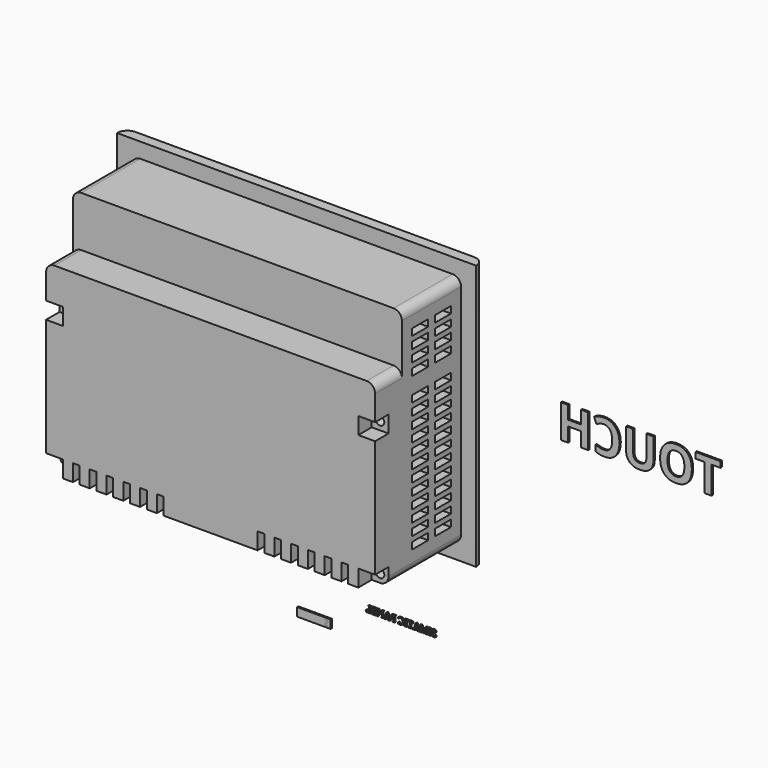
from build123d import *

# Parameters (mm, degrees)
F0_W          = 214
F0_H          = 158
F1_DEPTH      = 6.2
F2_W          = 196
F2_H          = 140
F3_DEPTH      = 44
F5_DEPTH      = 158
F6_W          = 196
F6_H          = 110
F7_DEPTH      = 20
F8_R          = 5
F9_W          = 12
F9_H          = 4
F10_DEPTH     = 10
F11_W         = 12
F11_H         = 4
F12_DEPTH     = 10
F13_W         = 10
F13_H         = 10
F14_DEPTH     = 10
F15_R         = 2.5
F16_DEPTH     = 20
F17_W         = 160
F17_H         = 120
F18_DEPTH     = 2
F19_W         = 140
F19_H         = 80
F20_DEPTH     = 2
F21_W         = 140
F21_H         = 80
F22_DEPTH     = 2
F23_W         = 4
F23_H         = 12
F24_DEPTH     = 10
F25_TEXT_SIZE = 5.5555555556
F26_DEPTH     = 1
F27_TEXT_SIZE = 27.7777777778
F28_DEPTH     = 1
F29_TEXT_SIZE = 4.1666666667
F30_DEPTH     = 1
F31_W         = 20
F31_H         = 5
F32_DEPTH     = 1


# Not quite as in the source:
# - Text() gives the source's letters only with a copy of the font that has no kerning and outlines rounded to 1/6400 em; it was checked with that copy


with BuildPart() as f1:
    # F0 (on Front) → F1 (new body)
    with BuildSketch(Plane.XZ):
        Rectangle(F0_W, F0_H)
    extrude(amount=-F1_DEPTH)

    # F2 (on face) → F3 (join)
    with BuildSketch(Plane.XZ):
        Rectangle(F2_W, F2_H)
    extrude(amount=F3_DEPTH)

    # F4 (on face) → F5 (cut)
    with BuildSketch(Plane.XY.offset(79)):
        with BuildLine():
            Line((107, 6.2), (100.8, 6.2))
            ThreePointArc((100.8, 6.2), (105.1840620434, 4.3840620434), (107, 0))
            Line((107, 0), (107, 6.2))
        make_face()
        with BuildLine():
            ThreePointArc((-107, 0), (-105.1840620434, 4.3840620434), (-100.8, 6.2))
            Line((-100.8, 6.2), (-107, 6.2))
            Line((-107, 6.2), (-107, 0))
        make_face()
    extrude(amount=-F5_DEPTH, mode=Mode.SUBTRACT)

    # F6 (on face) → F7 (join)
    with BuildSketch(Plane.XZ.offset(44)):
        with Locations((0, -15)):
            Rectangle(F6_W, F6_H)
    extrude(amount=F7_DEPTH)

    # F8
    f8_edges = [f1.edges().sort_by_distance(p)[0] for p in [
        (-98, -32, -70),
        (98, -32, -70),
        (98, -22, 70),
        (98, -54, 40),
        (-98, -22, 70),
        (-98, -54, 40),
    ]]
    fillet(f8_edges, radius=F8_R)

    # F9 (on face) → F10 (cut)
    with BuildSketch(Plane(origin=(-98, 0, 0), x_dir=(0, -1, 0), z_dir=(-1, 0, 0))):
        with Locations((13.5, -56)):
            Rectangle(F9_W, F9_H)
        with Locations((13.5, -49)):
            Rectangle(F9_W, F9_H)
        with Locations((13.5, -42)):
            Rectangle(F9_W, F9_H)
        with Locations((13.5, -35)):
            Rectangle(F9_W, F9_H)
        with Locations((13.5, -28)):
            Rectangle(F9_W, F9_H)
        with Locations((13.5, -21)):
            Rectangle(F9_W, F9_H)
        with Locations((13.5, -14)):
            Rectangle(F9_W, F9_H)
        with Locations((13.5, -7)):
            Rectangle(F9_W, F9_H)
        with Locations((13.5, 0)):
            Rectangle(F9_W, F9_H)
        with Locations((13.5, 7)):
            Rectangle(F9_W, F9_H)
        with Locations((13.5, 14)):
            Rectangle(F9_W, F9_H)
        with Locations((13.5, 21)):
            Rectangle(F9_W, F9_H)
        with Locations((13.5, 35)):
            Rectangle(F9_W, F9_H)
        with Locations((13.5, 42)):
            Rectangle(F9_W, F9_H)
        with Locations((13.5, 49)):
            Rectangle(F9_W, F9_H)
        with Locations((13.5, 56)):
            Rectangle(F9_W, F9_H)
        with Locations((30.5, 56)):
            Rectangle(F9_W, F9_H)
        with Locations((30.5, 49)):
            Rectangle(F9_W, F9_H)
        with Locations((30.5, 42)):
            Rectangle(F9_W, F9_H)
        with Locations((30.5, 35)):
            Rectangle(F9_W, F9_H)
        with Locations((30.5, 21)):
            Rectangle(F9_W, F9_H)
        with Locations((30.5, 14)):
            Rectangle(F9_W, F9_H)
        with Locations((30.5, 7)):
            Rectangle(F9_W, F9_H)
        with Locations((30.5, 0)):
            Rectangle(F9_W, F9_H)
        with Locations((30.5, -7)):
            Rectangle(F9_W, F9_H)
        with Locations((30.5, -14)):
            Rectangle(F9_W, F9_H)
        with Locations((30.5, -21)):
            Rectangle(F9_W, F9_H)
        with Locations((30.5, -28)):
            Rectangle(F9_W, F9_H)
        with Locations((30.5, -35)):
            Rectangle(F9_W, F9_H)
        with Locations((30.5, -42)):
            Rectangle(F9_W, F9_H)
        with Locations((30.5, -49)):
            Rectangle(F9_W, F9_H)
        with Locations((30.5, -56)):
            Rectangle(F9_W, F9_H)
    extrude(amount=-F10_DEPTH, mode=Mode.SUBTRACT)

    # F11 (on face) → F12 (cut)
    with BuildSketch(Plane.YZ.offset(98)):
        with Locations((-13.5, 56)):
            Rectangle(F11_W, F11_H)
        with Locations((-13.5, 49)):
            Rectangle(F11_W, F11_H)
        with Locations((-13.5, 42)):
            Rectangle(F11_W, F11_H)
        with Locations((-13.5, 35)):
            Rectangle(F11_W, F11_H)
        with Locations((-30.5, 56)):
            Rectangle(F11_W, F11_H)
        with Locations((-30.5, 49)):
            Rectangle(F11_W, F11_H)
        with Locations((-30.5, 42)):
            Rectangle(F11_W, F11_H)
        with Locations((-30.5, 35)):
            Rectangle(F11_W, F11_H)
        with Locations((-13.5, 21)):
            Rectangle(F11_W, F11_H)
        with Locations((-13.5, 14)):
            Rectangle(F11_W, F11_H)
        with Locations((-13.5, 7)):
            Rectangle(F11_W, F11_H)
        with Locations((-13.5, 0)):
            Rectangle(F11_W, F11_H)
        with Locations((-13.5, -7)):
            Rectangle(F11_W, F11_H)
        with Locations((-13.5, -14)):
            Rectangle(F11_W, F11_H)
        with Locations((-13.5, -21)):
            Rectangle(F11_W, F11_H)
        with Locations((-13.5, -28)):
            Rectangle(F11_W, F11_H)
        with Locations((-13.5, -35)):
            Rectangle(F11_W, F11_H)
        with Locations((-13.5, -42)):
            Rectangle(F11_W, F11_H)
        with Locations((-13.5, -49)):
            Rectangle(F11_W, F11_H)
        with Locations((-13.5, -56)):
            Rectangle(F11_W, F11_H)
        with Locations((-30.5, 21)):
            Rectangle(F11_W, F11_H)
        with Locations((-30.5, 14)):
            Rectangle(F11_W, F11_H)
        with Locations((-30.5, 7)):
            Rectangle(F11_W, F11_H)
        with Locations((-30.5, 0)):
            Rectangle(F11_W, F11_H)
        with Locations((-30.5, -7)):
            Rectangle(F11_W, F11_H)
        with Locations((-30.5, -14)):
            Rectangle(F11_W, F11_H)
        with Locations((-30.5, -21)):
            Rectangle(F11_W, F11_H)
        with Locations((-30.5, -28)):
            Rectangle(F11_W, F11_H)
        with Locations((-30.5, -35)):
            Rectangle(F11_W, F11_H)
        with Locations((-30.5, -42)):
            Rectangle(F11_W, F11_H)
        with Locations((-30.5, -49)):
            Rectangle(F11_W, F11_H)
        with Locations((-30.5, -56)):
            Rectangle(F11_W, F11_H)
    extrude(amount=-F12_DEPTH, mode=Mode.SUBTRACT)

    # F13 (on face) → F14 (cut)
    with BuildSketch(Plane.XZ.offset(64)):
        with BuildLine():
            Line((88, -70), (93, -70))
            ThreePointArc((93, -70), (96.5355339059, -68.5355339059), (98, -65))
            Line((98, -65), (98, -60))
            Line((98, -60), (88, -60))
            Line((88, -60), (88, -70))
        make_face()
        with BuildLine():
            Line((-93, -70), (-88, -70))
            Line((-88, -70), (-88, -60))
            Line((-88, -60), (-98, -60))
            Line((-98, -60), (-98, -65))
            ThreePointArc((-98, -65), (-96.5355339059, -68.5355339059), (-93, -70))
        make_face()
        with Locations((-93, 15)):
            Rectangle(F13_W, F13_H)
        with Locations((93, 15)):
            Rectangle(F13_W, F13_H)
    extrude(amount=-F14_DEPTH, mode=Mode.SUBTRACT)

    # F15 (on face) → F16 (cut)
    with BuildSketch(Plane.XZ.offset(54)):
        with Locations((93, -65)):
            Circle(F15_R)
        with Locations((93, 15)):
            Circle(F15_R)
        with Locations((-93, -65)):
            Circle(F15_R)
        with Locations((-93, 15)):
            Circle(F15_R)
    extrude(amount=-F16_DEPTH, mode=Mode.SUBTRACT)

    # F17 (on face) → F18 (cut)
    with BuildSketch(Plane(origin=(0, 6.2, 0), x_dir=(-1, 0, 0), z_dir=(0, 1, 0))):
        Rectangle(F17_W, F17_H)
    extrude(amount=-F18_DEPTH, mode=Mode.SUBTRACT)

    # F19 (on face) → F20 (join)
    with BuildSketch(Plane(origin=(0, 4.2, 0), x_dir=(-1, 0, 0), z_dir=(0, 1, 0))):
        with Locations((0, -10)):
            Rectangle(F19_W, F19_H)
        Polygon((62.5, 45), (62.5, 48.5), (55.5, 48.5), (55.5, 45), (55.5, 41.5), (62.5, 41.5), align=None)
        Polygon((40.5, 45), (40.5, 48.5), (33.5, 48.5), (33.5, 45), (33.5, 41.5), (40.5, 41.5), align=None)
        Polygon((18.5, 45), (18.5, 48.5), (11.5, 48.5), (11.5, 45), (11.5, 41.5), (18.5, 41.5), align=None)
        Polygon((-10.5, 48.5), (-10.5, 45), (-10.5, 41.5), (-3.5, 41.5), (-3.5, 45), (-3.5, 48.5), align=None)
        Polygon((-32.5, 48.5), (-32.5, 45), (-32.5, 41.5), (-25.5, 41.5), (-25.5, 45), (-25.5, 48.5), align=None)
        Polygon((-47.5, 45), (-47.5, 48.5), (-54.5, 48.5), (-54.5, 45), (-54.5, 41.5), (-47.5, 41.5), align=None)
    extrude(amount=F20_DEPTH)

    # F23 (on face) → F24 (cut)
    with BuildSketch(Plane(origin=(0, 0, -70), x_dir=(1, 0, 0), z_dir=(0, 0, -1))):
        with Locations((80, 58)):
            Rectangle(F23_W, F23_H)
        with Locations((70, 58)):
            Rectangle(F23_W, F23_H)
        with Locations((60, 58)):
            Rectangle(F23_W, F23_H)
        with Locations((50, 58)):
            Rectangle(F23_W, F23_H)
        with Locations((40, 58)):
            Rectangle(F23_W, F23_H)
        with Locations((30, 58)):
            Rectangle(F23_W, F23_H)
        with Locations((-30, 58)):
            Rectangle(F23_W, F23_H)
        with Locations((-40, 58)):
            Rectangle(F23_W, F23_H)
        with Locations((-50, 58)):
            Rectangle(F23_W, F23_H)
        with Locations((-60, 58)):
            Rectangle(F23_W, F23_H)
        with Locations((-70, 58)):
            Rectangle(F23_W, F23_H)
        with Locations((-80, 58)):
            Rectangle(F23_W, F23_H)
    extrude(amount=-F24_DEPTH, mode=Mode.SUBTRACT)


with BuildPart() as f22:
    # F21 (on face) → F22 (new body)
    with BuildSketch(Plane(origin=(0, 4.2, 0), x_dir=(-1, 0, 0), z_dir=(0, 1, 0))):
        Polygon((-80, -60), (80, -60), (80, 60), (62.5, 60), (62.5, 48.5), (62.5, 41.5), (55.5, 41.5), (55.5, 45), (47.5, 45), (47.5, 60), (40.5, 60), (40.5, 48.5), (40.5, 41.5), (33.5, 41.5), (33.5, 45), (25.5, 45), (25.5, 60), (18.5, 60), (18.5, 48.5), (18.5, 41.5), (11.5, 41.5), (11.5, 45), (3.5, 45), (3.5, 60), (-3.5, 60), (-3.5, 48.5), (-3.5, 41.5), (-10.5, 41.5), (-10.5, 45), (-18.5, 45), (-18.5, 60), (-25.5, 60), (-25.5, 48.5), (-25.5, 41.5), (-32.5, 41.5), (-32.5, 45), (-40.5, 45), (-40.5, 60), (-47.5, 60), (-47.5, 48.5), (-47.5, 41.5), (-54.5, 41.5), (-54.5, 45), (-62.5, 45), (-62.5, 60), (-80, 60), align=None)
        with Locations((0, -10)):
            Rectangle(F21_W, F21_H, mode=Mode.SUBTRACT)
    extrude(amount=F22_DEPTH)


with BuildPart() as f26:
    # F25 (on face) → F26 (new body)
    with BuildSketch(Plane(origin=(0, 6.2, 0), x_dir=(-1, 0, 0), z_dir=(0, 1, 0))):
        with Locations((-78.0516723032, -128.1266016682)):
            Text('SIMATIC PANEL', F25_TEXT_SIZE, font='Tinos', text_align=(TextAlign.LEFT, TextAlign.BOTTOM))
    extrude(amount=F26_DEPTH)


with BuildPart() as f28:
    # F27 (on face) → F28 (new body)
    with BuildSketch(Plane(origin=(0, 6.2, 0), x_dir=(-1, 0, 0), z_dir=(0, 1, 0))):
        with Locations((-248.2098141666, -0.1914162343)):
            Text('TOUCH', F27_TEXT_SIZE, font='Open Sans', font_style=FontStyle.BOLD, text_align=(TextAlign.LEFT, TextAlign.BOTTOM))
    extrude(amount=F28_DEPTH)


with BuildPart() as f30:
    # F29 (on face) → F30 (new body)
    with BuildSketch(Plane(origin=(0, 6.2, 0), x_dir=(-1, 0, 0), z_dir=(0, 1, 0))):
        with Locations((-14.0405010352, -142.9610185915)):
            Text('SIAMENS', F29_TEXT_SIZE, font='Open Sans', text_align=(TextAlign.LEFT, TextAlign.BOTTOM))
    extrude(amount=F30_DEPTH)


with BuildPart() as f32:
    # F31 (on face) → F32 (new body)
    with BuildSketch(Plane.XZ.offset(-6.2)):
        with Locations((5.3755551804, -141.4015716314)):
            Rectangle(F31_W, F31_H)
        with BuildLine():
            Line((13.8250062435, -142.5319821332), (13.8250062435, -142.8653154665))
            add(Edge.make_bspline(
                [(13.8250062435, -142.8653154665), (13.5398499935, -143.0020342165), (12.5229229102, -143.0020342165), (11.9532614519, -142.5619300499), (11.9532614519, -141.8646644249), (12.3048239519, -141.4818519249), (12.7729229102, -141.3151852582)],
                knots=[0, 0, 0, 1, 1.9236453202, 2.8472906404, 3.5641496949, 4.2810087494, 4.2810087494, 4.2810087494], degree=2))
            add(Edge.make_bspline(
                [(12.7729229102, -141.3151852582), (13.0515687435, -141.2155758832), (13.3224020769, -141.0508623415), (13.4363343685, -140.8529456749), (13.4363343685, -140.4890133832), (13.1270895769, -140.2533362999), (12.5046937435, -140.2533362999), (12.1362041602, -140.4076331749)],
                knots=[0, 0, 0, 1, 2, 3, 4.358649789, 5.7172995781, 7.4365388846, 7.4365388846, 7.4365388846], degree=2))
            Line((12.1362041602, -140.4076331749), (12.0281312435, -140.1068519249))
            add(Edge.make_bspline(
                [(12.0281312435, -140.1068519249), (12.4005270769, -139.9440915082), (13.2696677019, -139.9440915082), (13.7859437435, -140.3509925499), (13.7859437435, -141.0222165082), (13.4298239519, -141.4291175499), (13.0151104102, -141.5775550499)],
                knots=[0, 0, 0, 1, 1.9603524229, 2.9207048458, 3.8355860366, 4.7504672273, 4.7504672273, 4.7504672273], degree=2))
            add(Edge.make_bspline(
                [(13.0151104102, -141.5775550499), (12.7182354102, -141.6830237999), (12.4272197852, -141.8503415082), (12.3028708269, -142.0476071332), (12.3028708269, -142.4362790082), (12.6531312435, -142.6986487999), (13.2104229102, -142.6986487999), (13.6414124935, -142.6088050499), (13.8250062435, -142.5319821332)],
                knots=[0, 0, 0, 1, 2, 3, 4.5189873418, 6.0379746835, 6.967675034, 7.8973753844, 7.8973753844, 7.8973753844], degree=2))
        make_face(mode=Mode.SUBTRACT)
    extrude(amount=-F32_DEPTH)


solid = Compound([f1.part, f22.part, f26.part, f28.part, f30.part, f32.part])
